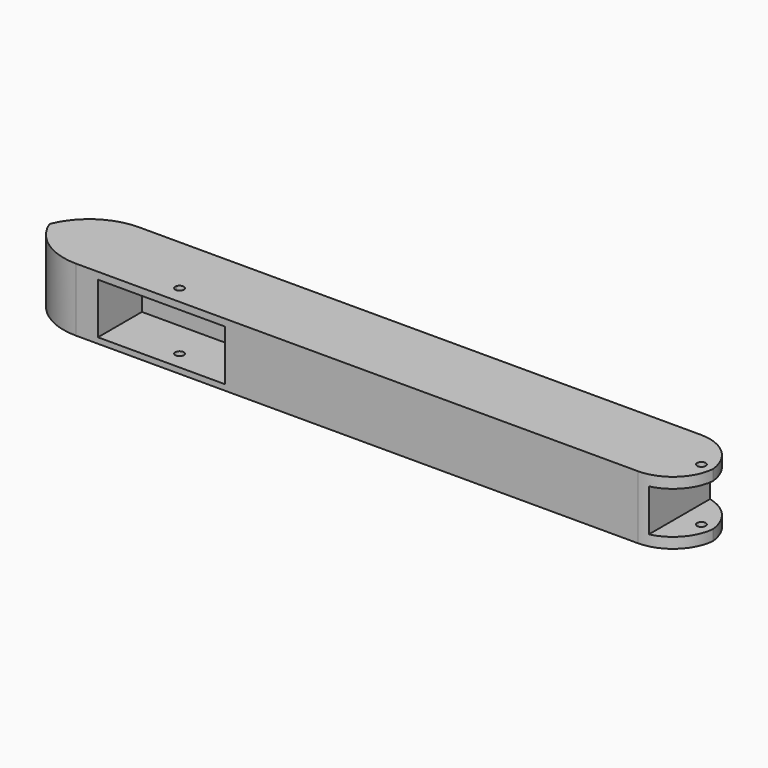
from build123d import *

# Parameters (mm, degrees)
F0_W         = 1500
F0_H         = 150
F1_DEPTH     = 56.30659
F2_W         = 1500
F2_H         = 150
F2_W_2       = 300.6279
F2_H_2       = 120
F3_DEPTH     = 130
F6_D         = 20
F6_DEPTH     = 16.486247664
F7_D         = 20
F8_T1_DEPTH  = 887.8761290407
F9_W         = 186.30659
F9_H         = 25
F10_DEPTH    = 80
F11_T1_DEPTH = 543.3223571193
F11_T3_DEPTH = 543.3223571193
F13_D        = 20


# Not quite as in the source:
# - a fillet or chamfer that OpenCascade refuses, or shapes differently, is made with other operations: its cross-section is extruded or revolved along the edge and cut away or added
# - a feature names something its author has since deleted; it is built from what else it names


with BuildPart() as f1:
    # F0 (on Front) → F1 (new body)
    with BuildSketch(Plane.XZ):
        with Locations((295.444762387, 72.4433880299)):
            Rectangle(F0_W, F0_H)
    extrude(amount=F1_DEPTH)

    # F2 (on face) → F3 (join)
    with BuildSketch(Plane.XZ.offset(56.30659)):
        with Locations((295.444762387, 72.4433880299)):
            Rectangle(F2_W, F2_H)
        with Locations((-104.6067848625, 70.9581403659)):
            Rectangle(F2_W_2, F2_H_2, mode=Mode.SUBTRACT)
    extrude(amount=F3_DEPTH)

    # F6 (through all, one way)
    with BuildSketch(Plane(origin=(0, 0, 130.9581403659), x_dir=(1, 0, 0), z_dir=(0, 0, -1))):
        with Locations((-96.1152985692, 143.3657854795)):
            Circle(F6_D / 2)
    extrude(amount=-F6_DEPTH, mode=Mode.SUBTRACT)

    # F7 (through all)
    with Locations(Plane(origin=(0, 0, -2.5566119701), x_dir=(1, 0, 0), z_dir=(0, 0, -1))):
        with Locations((-96.1604490876, 143.5462683439)):
            Hole(F7_D / 2)

    # F8: fillet of radius 147.5752258081 on 2 edges, made by hand

    # F8_s2 → F8_t1 (cut)
    with BuildSketch(Plane.XY.offset(-371.4946764904)):
        with BuildLine():
            ThreePointArc((-454.555237613, -38.7313641919), (-411.331454709, -143.0828070959), (-306.9800118049, -186.30659))
            Line((-306.9800118049, -186.30659), (-454.555237613, -186.30659))
            Line((-454.555237613, -186.30659), (-454.555237613, -38.7313641919))
        make_face()
        with BuildLine():
            ThreePointArc((-306.9800118049, 0), (-411.331454709, -43.2237829041), (-454.555237613, -147.5752258081))
            Line((-454.555237613, -147.5752258081), (-454.555237613, 0))
            Line((-454.555237613, 0), (-306.9800118049, 0))
        make_face()
    extrude(amount=F8_T1_DEPTH, mode=Mode.SUBTRACT)

    # F9 (on face) → F10 (join)
    with BuildSketch(Plane.YZ.offset(1045.444762387)):
        with Locations((-93.153295, 134.9433880299)):
            Rectangle(F9_W, F9_H)
        with Locations((-93.153295, 9.9433880299)):
            Rectangle(F9_W, F9_H)
    extrude(amount=F10_DEPTH)

    # F11: fillet of radius 103.6644714239 on 4 edges, made by hand

    # F11_s2 → F11_t1 (cut)
    with BuildSketch(Plane.XY.offset(-136.7177905297)):
        with BuildLine():
            ThreePointArc((1125.444762387, -103.6644714239), (1095.082141675, -30.3626207119), (1021.7802909631, 0))
            Line((1021.7802909631, 0), (1125.444762387, 0))
            Line((1125.444762387, 0), (1125.444762387, -103.6644714239))
        make_face()
        with BuildLine():
            ThreePointArc((1021.7802909631, -186.30659), (1095.082141675, -155.9439692881), (1125.444762387, -82.6421185761))
            Line((1125.444762387, -82.6421185761), (1125.444762387, -186.30659))
            Line((1125.444762387, -186.30659), (1021.7802909631, -186.30659))
        make_face()
    extrude(amount=F11_T1_DEPTH, mode=Mode.SUBTRACT)

    # F11_s4 → F11_t3 (cut)
    with BuildSketch(Plane.XY.offset(-261.7177905297)):
        with BuildLine():
            ThreePointArc((1125.444762387, -103.6644714239), (1095.082141675, -30.3626207119), (1021.7802909631, 0))
            Line((1021.7802909631, 0), (1125.444762387, 0))
            Line((1125.444762387, 0), (1125.444762387, -103.6644714239))
        make_face()
        with BuildLine():
            ThreePointArc((1021.7802909631, -186.30659), (1095.082141675, -155.9439692881), (1125.444762387, -82.6421185761))
            Line((1125.444762387, -82.6421185761), (1125.444762387, -186.30659))
            Line((1125.444762387, -186.30659), (1021.7802909631, -186.30659))
        make_face()
    extrude(amount=F11_T3_DEPTH, mode=Mode.SUBTRACT)

    # F13 (through all)
    with Locations(Plane(origin=(0, 0, -2.5566119701), x_dir=(1, 0, 0), z_dir=(0, 0, -1))):
        with Locations((1096.6192483902, 92.0223891735)):
            Hole(F13_D / 2)


solid = f1.part
